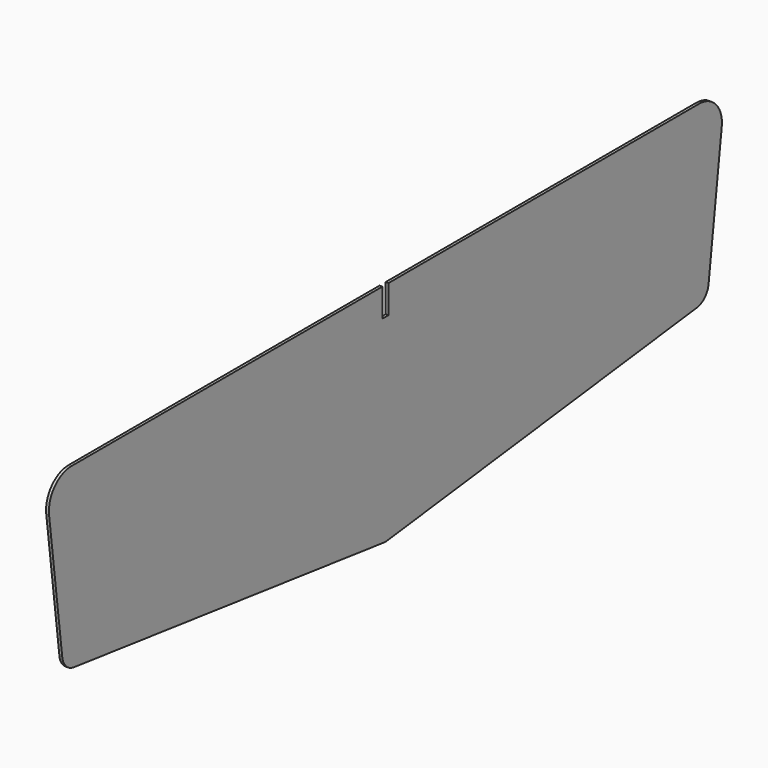
from build123d import *

# Parameters (mm, degrees)
F1_DEPTH = 1


# Not quite as in the source:
# - ends of sketch curves that miss each other by under 0.0002 mm in the source are joined


with BuildPart() as f1:
    # F0 (on Right) → F1 (new body)
    with BuildSketch(Plane.YZ):
        with BuildLine():
            Line((-17.710118, -7.110515), (-155.042295, -7.110515))
            ThreePointArc((-155.042295, -7.110515), (-162.539076635, -10.4924892282), (-164.9650738133, -18.3508619767))
            Line((-164.9650738133, -18.3508619767), (-159.139913, -64.952155))
            ThreePointArc((-159.139913, -64.952155), (-157.4251457547, -68.4543233257), (-153.91996093, -70.1629154318))
            Line((-153.91996093, -70.1629154318), (-16.370118, -87.110515))
            Line((-16.370118, -87.110515), (121.179726, -70.162916))
            ThreePointArc((121.179726, -70.162916), (124.6849107108, -68.4543233695), (126.3996771834, -64.9521550229))
            Line((126.3996771834, -64.9521550229), (132.224839, -18.350862))
            ThreePointArc((132.224839, -18.350862), (129.798841635, -10.4924892282), (122.30206, -7.110515))
            Line((122.30206, -7.110515), (-15.030118, -7.110515))
            Line((-15.030118, -7.110515), (-15.030118, -17.110515))
            Line((-15.030118, -17.110515), (-17.710118, -17.110515))
            Line((-17.710118, -17.110515), (-17.710118, -7.110515))
        make_face()
    extrude(amount=F1_DEPTH)


solid = f1.part
